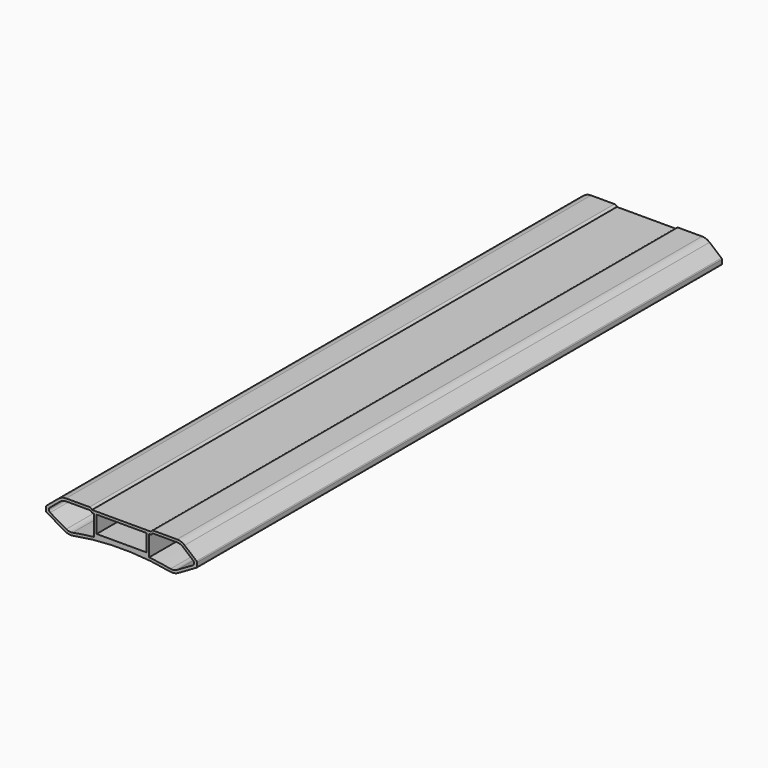
from build123d import *

# Parameters (mm, degrees)
F1_DEPTH    = 250
F2_W        = 38
F2_H        = 13
F3_DEPTH    = 250
F4_T1_DEPTH = 509.3674969976
F5_R        = 9
F6_R        = 1
F8_DEPTH    = 250


# Not quite as in the source:
# - a fillet or chamfer that OpenCascade refuses, or shapes differently, is made with other operations: its cross-section is extruded or revolved along the edge and cut away or added


with BuildPart() as f1:
    # F0 (on Front) → F1 (new body, symmetric)
    with BuildSketch(Plane.XZ):
        with BuildLine():
            Line((22.5, 0), (0, 0))
            Line((0, 0), (-22.5, 0))
            Line((-22.5, 0), (-22.5, 1.3))
            Line((-22.5, 1.3), (-45.5824640741, 1.3))
            Line((-45.5824640741, 1.3), (-57.5, -8.7))
            Line((-57.5, -8.7), (-57.5, -12.7))
            Line((-57.5, -12.7), (-40.1794919243, -22.7))
            ThreePointArc((-40.1794919243, -22.7), (0, -18.6224551416), (40.1794919243, -22.7))
            Line((40.1794919243, -22.7), (57.5, -12.7))
            Line((57.5, -12.7), (57.5, -8.7))
            Line((57.5, -8.7), (45.5824640741, 1.3))
            Line((45.5824640741, 1.3), (22.5, 1.3))
            Line((22.5, 1.3), (22.5, 0))
        make_face()
    extrude(amount=F1_DEPTH, both=True)

    # F2 (on Front) → F3 (cut, symmetric)
    with BuildSketch(Plane.XZ):
        with Locations((0, -8.5)):
            Rectangle(F2_W, F2_H)
    extrude(amount=F3_DEPTH, both=True, mode=Mode.SUBTRACT)

    # F4: fillet of radius 2 on 2 edges, made by hand

    # F4_s2 → F4_t1 (cut)
    with BuildSketch(Plane.XZ.offset(-254.6837484988)):
        with BuildLine():
            ThreePointArc((24.3734993995, 1.3), (23.2333239744, 0.9431676725), (22.5, 0))
            Line((22.5, 0), (22.5, 1.3))
            Line((22.5, 1.3), (24.3734993995, 1.3))
        make_face()
        with BuildLine():
            ThreePointArc((-24.3734993995, 1.3), (-23.2333239744, 0.9431676725), (-22.5, 0))
            Line((-22.5, 0), (-22.5, 1.3))
            Line((-22.5, 1.3), (-24.3734993995, 1.3))
        make_face()
    extrude(amount=F4_T1_DEPTH, mode=Mode.SUBTRACT)

    # F5
    f5_edges = [f1.edges().sort_by_distance(p)[0] for p in [
        (45.582464, 0, 1.3),
        (-45.582464, 0, 1.3),
        (40.179492, 0, -22.7),
        (-40.179492, 0, -22.7),
    ]]
    fillet(f5_edges, radius=F5_R)

    # F6
    f6_edges = [f1.edges().sort_by_distance(p)[0] for p in [
        (57.5, 0, -8.7),
        (57.5, 0, -12.7),
        (-57.5, 0, -8.7),
        (-57.5, 0, -12.7),
    ]]
    fillet(f6_edges, radius=F6_R)

    # F7 (on Front) → F8 (cut, symmetric)
    with BuildSketch(Plane.XZ):
        with BuildLine():
            ThreePointArc((-42.1022690923, -19.2804830077), (-39.7790673433, -20.1186780608), (-37.3093701274, -20.0978700124))
            ThreePointArc((-37.3093701274, -20.0978700124), (-29.1789785809, -18.7410222645), (-21, -17.7170047426))
            Line((-21, -17.7170047426), (-21, -2))
            Line((-21, -2), (-22.5, -2))
            ThreePointArc((-22.5, -2), (-23.2333239744, -1.0568323275), (-24.3734993995, -0.7))
            Line((-24.3734993995, -0.7), (-42.3067319657, -0.7))
            ThreePointArc((-42.3067319657, -0.7), (-44.7008729689, -1.1221516545), (-46.8062452335, -2.3376888982))
            Line((-46.8062452335, -2.3376888982), (-54.6622869129, -8.9296905739))
            ThreePointArc((-54.6622869129, -8.9296905739), (-55.3691010897, -10.6360909457), (-54.3767116936, -12.1938302677))
            Line((-54.3767116936, -12.1938302677), (-42.1022690923, -19.2804830077))
        make_face()
        with BuildLine():
            Line((42.3067319657, -0.7), (24.3734993995, -0.7))
            ThreePointArc((24.3734993995, -0.7), (23.2333239744, -1.0568323275), (22.5, -2))
            Line((22.5, -2), (21, -2))
            Line((21, -2), (21, -17.7170047426))
            ThreePointArc((21, -17.7170047426), (29.1789785809, -18.7410222645), (37.3093701274, -20.0978700124))
            ThreePointArc((37.3093701274, -20.0978700124), (39.7790673433, -20.1186780608), (42.1022690923, -19.2804830077))
            Line((42.1022690923, -19.2804830077), (54.3767116936, -12.1938302677))
            ThreePointArc((54.3767116936, -12.1938302677), (55.3691010897, -10.6360909457), (54.6622869129, -8.9296905739))
            Line((54.6622869129, -8.9296905739), (46.8062452335, -2.3376888982))
            ThreePointArc((46.8062452335, -2.3376888982), (44.7008729689, -1.1221516545), (42.3067319657, -0.7))
        make_face()
    extrude(amount=F8_DEPTH, both=True, mode=Mode.SUBTRACT)


solid = f1.part
